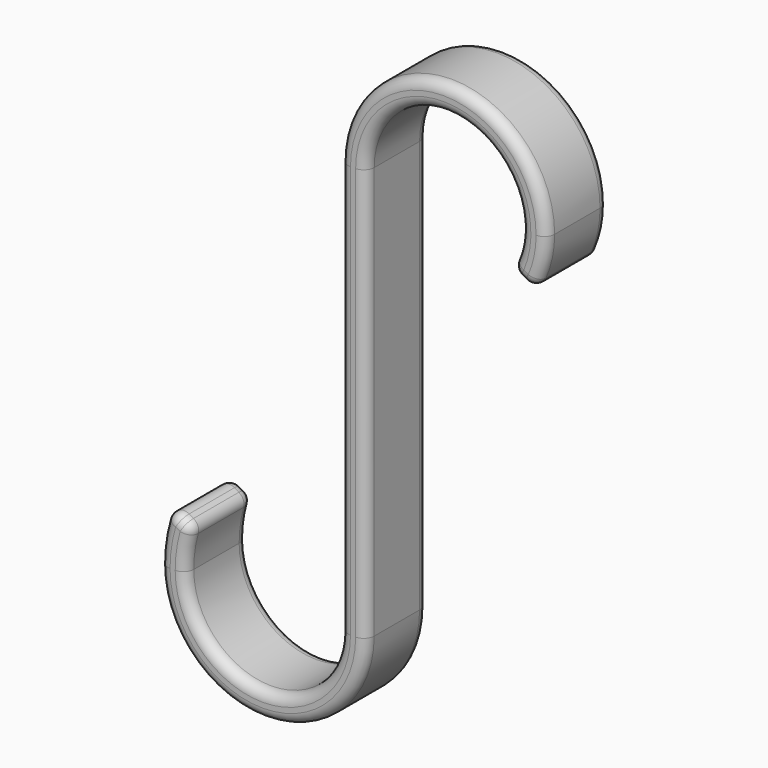
from build123d import *

# Parameters (mm, degrees)
F1_DEPTH = 19.05
F2_R     = 2.54


# Not quite as in the source:
# - a feature names something its author has since deleted; it is built from what else it names


with BuildPart() as f1:
    # F0 (on Front) → F1 (new body)
    with BuildSketch(Plane.XZ):
        with BuildLine():
            ThreePointArc((13.97, 0), (-11.43, 25.4), (-36.83, 0))
            Line((-36.83, 0), (-36.83, -101.6))
            ThreePointArc((-36.83, -101.6), (-55.88, -120.65), (-74.93, -101.6))
            ThreePointArc((-74.93, -101.6), (-74.5044281022, -96.5179462529), (-73.2395664242, -91.577449652))
            Line((-73.2395664242, -91.577449652), (-78.7388277382, -88.402449652))
            ThreePointArc((-78.7388277382, -88.402449652), (-80.638925247, -94.8800131761), (-81.28, -101.6))
            ThreePointArc((-81.28, -101.6), (-55.88, -127), (-30.48, -101.6))
            Line((-30.48, -101.6), (-30.48, 0))
            ThreePointArc((-30.48, 0), (-6.4994971908, 18.4008869908), (5.0677839421, -9.525))
            Line((5.0677839421, -9.525), (10.5670452561, -12.7))
            ThreePointArc((10.5670452561, -12.7), (13.1045159877, -6.5740037456), (13.97, 0))
        make_face()
    extrude(amount=F1_DEPTH)

    # F2
    f2_edges = [f1.edges().sort_by_distance(p)[0] for p in [
        (-73.239566, -9.525, -91.57745),
        (-78.738828, -9.525, -88.40245),
        (-75.989197, 0, -89.98995),
        (-75.989197, -19.05, -89.98995),
        (5.067784, -9.525, -9.525),
        (10.567045, -9.525, -12.7),
        (7.817415, 0, -11.1125),
        (7.817415, -19.05, -11.1125),
        (-30.48, 0, -50.8),
        (-6.499497, 0, 18.400887),
        (-4.855996, 0, 24.534516),
        (-36.83, 0, -50.8),
        (-55.88, 0, -120.65),
        (-74.504428, 0, -96.517946),
        (-80.638925, 0, -94.880013),
        (-55.88, 0, -127),
        (-30.48, -19.05, -50.8),
        (-6.499497, -19.05, 18.400887),
        (-4.855996, -19.05, 24.534516),
        (-36.83, -19.05, -50.8),
        (-55.88, -19.05, -120.65),
        (-74.504428, -19.05, -96.517946),
        (-80.638925, -19.05, -94.880013),
        (-55.88, -19.05, -127),
    ]]
    fillet(f2_edges, radius=F2_R)


solid = f1.part
